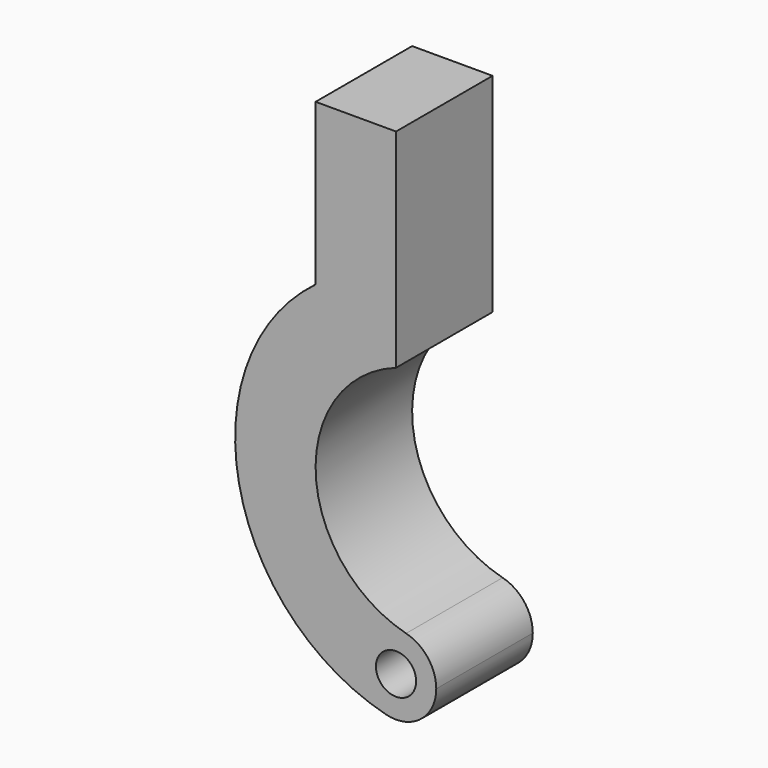
from build123d import *

# Parameters (mm, degrees)
F1_DEPTH = 15
F2_R     = 4.99999
F3_R     = 2.5
F4_DEPTH = 15.001


# Not quite as in the source:
# - a fillet or chamfer is up to 0.001 mm smaller than in the source, because OpenCascade refuses the exact size


with BuildPart() as f1:
    # F0 (on Front) → F1 (new body)
    with BuildSketch(Plane.XZ):
        with BuildLine():
            Line((-15, 40), (-15, 20))
            ThreePointArc((-15, 20), (-23.7170824513, -7.9056941504), (0, -25))
            Line((0, -25), (0, -15))
            ThreePointArc((0, -15), (-14.7839783948, -2.5365296809), (-5, 14.1421356237))
            Line((-5, 14.1421356237), (-5, 40))
            Line((-5, 40), (-15, 40))
        make_face()
    extrude(amount=F1_DEPTH)

    # F2 (radius 5 in the source; OpenCascade refuses exactly that, so slightly less here)
    f2_edges = [f1.edges().sort_by_distance(p)[0] for p in [
        (0, -7.5, -25),
        (0, -7.5, -15),
    ]]
    fillet(f2_edges, radius=F2_R)

    # F3 (on face) → F4 (cut, through all)
    with BuildSketch(Plane.XZ.offset(15)):
        with Locations((-5, -19.364916731)):
            Circle(F3_R)
    extrude(amount=-F4_DEPTH, mode=Mode.SUBTRACT)


solid = f1.part
